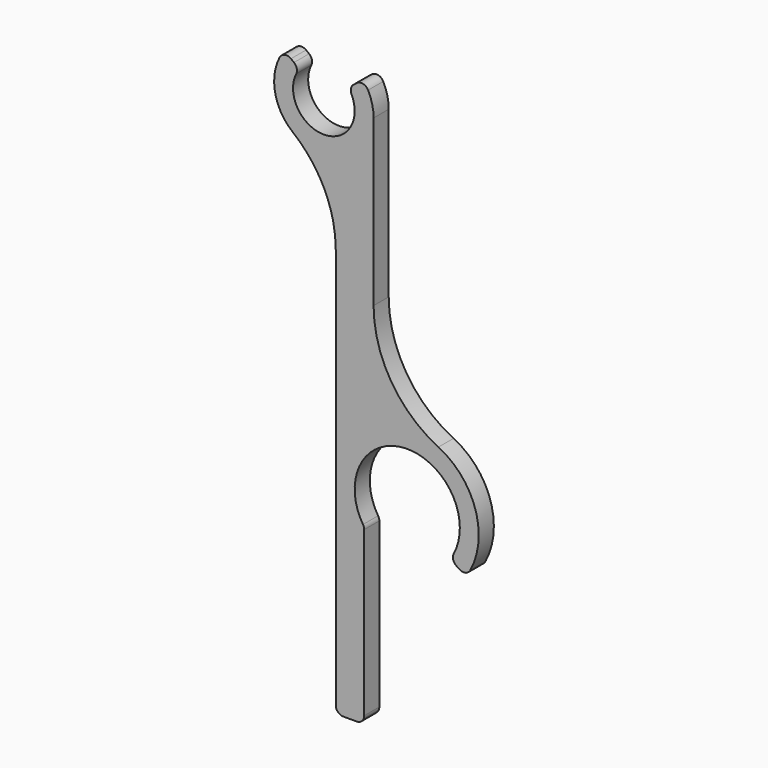
from build123d import *

# Parameters (mm, degrees)
F1_DEPTH = 5
F2_R     = 2
F3_R     = 30.3991713246


with BuildPart() as f1:
    # F0 (on Front) → F1 (new body)
    with BuildSketch(Plane.XZ):
        with BuildLine():
            ThreePointArc((8.4325112108, -10.0903545369), (5.9438997073, -11.7299853482), (3.15, -12.7671453348))
            Line((3.15, -12.7671453348), (3.15, -88.05))
            ThreePointArc((3.15, -88.05), (3.6076950345, -83.915826859), (4.9586124402, -79.9818855189))
            ThreePointArc((4.9586124402, -79.9818855189), (8.3605698088, -75.0189025389), (13.15, -71.3766679995))
            Line((13.15, -71.3766679995), (13.15, 0))
            ThreePointArc((13.15, 0), (11.91238898, -5.569334681), (8.4325112108, -10.0903545369))
        make_face()
        with BuildLine():
            ThreePointArc((4.9586124402, -79.9818855189), (3.6076950345, -83.915826859), (3.15, -88.05))
            ThreePointArc((3.15, -88.05), (4.0247496309, -93.7333396106), (6.5680263629, -98.890594647))
            Line((6.5680263629, -98.890594647), (10.6637865844, -96.0227124653))
            ThreePointArc((10.6637865844, -96.0227124653), (22.05, -74.15), (33.4362134156, -96.0227124653))
            Line((33.4362134156, -96.0227124653), (37.5319736371, -98.890594647))
            ThreePointArc((37.5319736371, -98.890594647), (36.1951275757, -75.5150342694), (13.15, -71.3766679995))
            ThreePointArc((13.15, -71.3766679995), (8.3605698088, -75.0189025389), (4.9586124402, -79.9818855189))
        make_face()
        with BuildLine():
            ThreePointArc((6.5680263629, -98.890594647), (4.0247496309, -93.7333396106), (3.15, -88.05))
            Line((3.15, -88.05), (3.15, -141.95))
            Line((3.15, -141.95), (10.6637865844, -141.95))
            Line((10.6637865844, -141.95), (10.6637865844, -103.1352293338))
            ThreePointArc((10.6637865844, -103.1352293338), (8.4492978203, -101.1736770845), (6.5680263629, -98.890594647))
        make_face()
        with BuildLine():
            Line((10.6637865844, -96.0227124653), (6.5680263629, -98.890594647))
            ThreePointArc((6.5680263629, -98.890594647), (8.4492978203, -101.1736770845), (10.6637865844, -103.1352293338))
            Line((10.6637865844, -103.1352293338), (10.6637865844, -96.0227124653))
        make_face()
        with BuildLine():
            ThreePointArc((-10.4325964248, 8.0052127915), (-12.666067706, -3.5345761935), (-4.7800799709, -12.2504422562))
            ThreePointArc((-4.7800799709, -12.2504422562), (-0.8550062548, -13.1221745265), (3.15, -12.7671453348))
            ThreePointArc((3.15, -12.7671453348), (5.9438997073, -11.7299853482), (8.4325112108, -10.0903545369))
            ThreePointArc((8.4325112108, -10.0903545369), (11.91238898, -5.569334681), (13.15, 0))
            ThreePointArc((13.15, 0), (12.4521312029, 4.2269289687), (10.4325964248, 8.0052127915))
            Line((10.4325964248, 8.0052127915), (6.4658297234, 4.9614056464))
            ThreePointArc((6.4658297234, 4.9614056464), (0, -8.15), (-6.4658297234, 4.9614056464))
            Line((-6.4658297234, 4.9614056464), (-10.4325964248, 8.0052127915))
        make_face()
    extrude(amount=F1_DEPTH)

    # F2
    f2_edges = [f1.edges().sort_by_distance(p)[0] for p in [
        (6.46583, -2.5, 4.961406),
        (-6.46583, -2.5, 4.961406),
        (-10.432596, -2.5, 8.005213),
        (10.663787, -2.5, -96.022712),
        (33.436213, -2.5, -96.022712),
        (37.531974, -2.5, -98.890595),
        (3.15, -2.5, -141.95),
        (10.663787, -2.5, -141.95),
        (10.432596, -2.5, 8.005213),
    ]]
    fillet(f2_edges, radius=F2_R)

    # F3
    f3_edges = [f1.edges().sort_by_distance(p)[0] for p in [
        (3.15, -2.5, -12.767145),
        (13.15, -2.5, -71.376668),
    ]]
    fillet(f3_edges, radius=F3_R)


solid = f1.part
